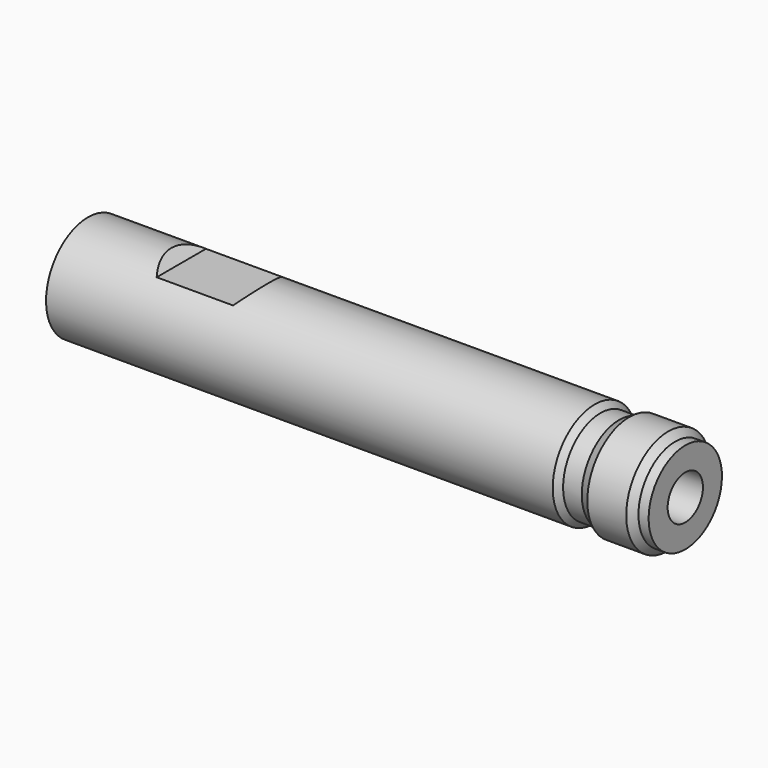
from build123d import *

# Parameters (mm, degrees)
F2_R     = 3.302
F3_DEPTH = 89.409
F5_DEPTH = 12.7


# Not quite as in the source:
# - a pattern or mirror of a feature is missing from the dataset's text; its kind, count and spacing are read off the source's solid


with BuildPart() as f1:
    # F0 (on Front) → F1 (revolve)
    with BuildSketch(Plane.XZ):
        Polygon((75.8444, 7.8486), (0, 7.8486), (0, 5.715), (11.43, 5.715), (11.43, 0), (89.408, 0), (89.408, 6.858), (87.884, 6.858), (86.868, 7.874), (81.0417931679, 7.874), (79.502, 6.985), (76.708, 6.985), align=None)
    revolve(axis=Axis((72.7860965579, 0, 0), (1, 0, 0)))

    # F2 (on face) → F3 (cut, through all)
    with BuildSketch(Plane.YZ.offset(89.408)):
        Circle(F2_R)
    extrude(amount=-F3_DEPTH, mode=Mode.SUBTRACT)

    # F4 (on Front) → F5 (cut, symmetric)
    with BuildSketch(Plane.XZ):
        Polygon((0, 20.32), (13.97, 6.35), (25.4, 6.35), (39.37, 20.32), align=None)
    f5 = extrude(amount=F5_DEPTH, both=True, mode=Mode.SUBTRACT)

    # F5_copies: F5 across plane
    add(f5.mirror(Plane(origin=(0, 0, 0), x_dir=(-1, 0, 0), z_dir=(0, 0, -1))), mode=Mode.SUBTRACT)


solid = f1.part
